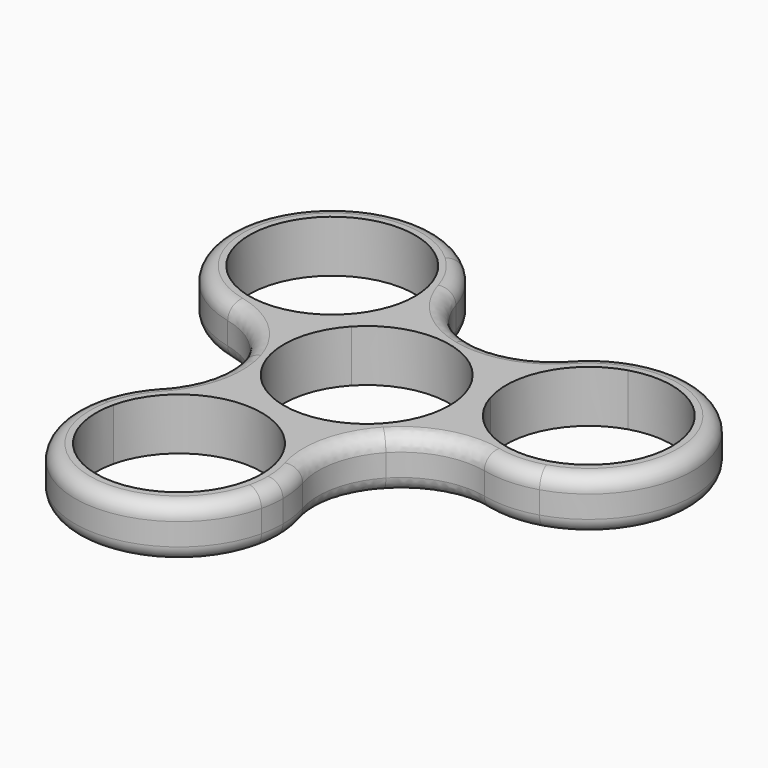
from build123d import *

# Parameters (mm, degrees)
F1_DEPTH = 7
F2_R     = 11.149
F3_R     = 2


# Not quite as in the source:
# - a fillet or chamfer is up to 0.001 mm smaller than in the source, because OpenCascade refuses the exact size


with BuildPart() as f1:
    # F0 (on Top) → F1 (new body)
    with BuildSketch(Plane.XY):
        with BuildLine():
            Line((-27.9345224248, 6.9415385111), (-25.9887218323, 9.0239313785))
            ThreePointArc((-25.9887218323, 9.0239313785), (-26.5231091537, 24.7833549146), (-10.7636856175, 25.317742236))
            Line((-10.7636856175, 25.317742236), (-8.8178850251, 27.4001351034))
            ThreePointArc((-8.8178850251, 27.4001351034), (-28.6055020211, 26.7291555071), (-27.9345224248, 6.9415385111))
        make_face()
        with BuildLine():
            ThreePointArc((-7.2262037249, 17.1708368072), (-8.0041138961, 13.0791070283), (-10.2292983588, 9.5583186329))
            ThreePointArc((-10.2292983588, 9.5583186329), (-7.8092966531, 11.6195906031), (-4.9866679164, 13.0817866934))
            ThreePointArc((-4.9866679164, 13.0817866934), (-4.5296608113, 15.1036528917), (-4.3762037249, 17.1708368072))
            ThreePointArc((-4.3762037249, 17.1708368072), (-4.3804864458, 17.5170994861), (-4.3933319882, 17.8631503155))
            ThreePointArc((-4.3933319882, 17.8631503155), (-7.4355430712, 22.246605973), (-8.8178850251, 27.4001351034))
            Line((-8.8178850251, 27.4001351034), (-10.7636856175, 25.317742236))
            ThreePointArc((-10.7636856175, 25.317742236), (-8.1487388167, 21.6117220288), (-7.2262037249, 17.1708368072))
        make_face()
        with BuildLine():
            Line((-10.2292982962, 9.5583186998), (-8.1469054287, 7.6125181074))
            ThreePointArc((-8.1469053912, 7.6125181475), (-6.2542997422, 10.166592106), (-4.9866679164, 13.0817866934))
            ThreePointArc((-4.9866679164, 13.0817866934), (-7.8092966531, 11.6195906031), (-10.2292983588, 9.5583186329))
        make_face()
        with BuildLine():
            ThreePointArc((-13.3895358085, 4.0890501138), (-10.5669070871, 5.5512461938), (-8.1469053912, 7.6125181475))
            Line((-8.1469054287, 7.6125181074), (-10.2292982962, 9.5583186998))
            ThreePointArc((-10.2292983588, 9.5583186329), (-12.1219039919, 7.0042446853), (-13.3895358085, 4.0890501138))
        make_face()
        with BuildLine():
            ThreePointArc((-13.3895358085, 4.0890501138), (-12.1219039919, 7.0042446853), (-10.2292983588, 9.5583186329))
            ThreePointArc((-10.2292983588, 9.5583186329), (-17.998334872, 6.0272415557), (-25.9887218323, 9.0239313785))
            Line((-25.9887218323, 9.0239313785), (-27.9345224248, 6.9415385111))
            ThreePointArc((-27.9345224248, 6.9415385111), (-22.699190816, 5.9114731141), (-18.11972388, 3.1731863583))
            ThreePointArc((-18.11972388, 3.1731863583), (-15.7149350018, 3.4261051335), (-13.3895358085, 4.0890501138))
        make_face()
        with BuildLine():
            ThreePointArc((-16.543965134, -21.9804963011), (-11.5813207167, -15.0379755337), (-3.1630976847, -13.6379915324))
            ThreePointArc((-3.1630976847, -13.6379915324), (-6.1582123683, -12.5728445638), (-8.8358256451, -10.8594744426))
            ThreePointArc((-8.8358256451, -10.8594744426), (-11.1358956381, -11.6055679238), (-13.2732759707, -12.7363122668))
            ThreePointArc((-13.2732759707, -12.7363122668), (-15.548354385, -17.5626721771), (-19.3202705541, -21.3365799911))
            Line((-19.3202705541, -21.3365799911), (-16.543965134, -21.9804963011))
        make_face()
        with BuildLine():
            Line((-3.1630976634, -13.6379915373), (-2.5191813534, -10.8616861172))
            ThreePointArc((-2.5191814257, -10.8616861004), (-5.6773771723, -10.4996785127), (-8.8358256451, -10.8594744426))
            ThreePointArc((-8.8358256451, -10.8594744426), (-6.1582123683, -12.5728445638), (-3.1630976847, -13.6379915324))
        make_face()
        with BuildLine():
            ThreePointArc((3.1535466283, -13.6402032119), (0.4759333083, -11.9268330695), (-2.5191814257, -10.8616861004))
            Line((-2.5191813534, -10.8616861172), (-3.1630976634, -13.6379915373))
            ThreePointArc((-3.1630976847, -13.6379915324), (-0.0049018926, -13.9999991418), (3.1535466283, -13.6402032119))
        make_face()
        with BuildLine():
            ThreePointArc((3.1535466283, -13.6402032119), (-0.0049018926, -13.9999991418), (-3.1630976847, -13.6379915324))
            ThreePointArc((-3.1630976847, -13.6379915324), (3.0473077962, -17.5630492175), (5.4677209832, -24.4996776545))
            ThreePointArc((5.4677209832, -24.4996776545), (5.3954080208, -25.7674906914), (5.1794071004, -27.0188590079))
            Line((5.1794071004, -27.0188590079), (7.9557125205, -27.662775318))
            ThreePointArc((7.9557125205, -27.662775318), (6.2301095174, -22.6138124491), (6.3118019427, -17.2787343688))
            ThreePointArc((6.3118019427, -17.2787343688), (4.8903734193, -15.3225854971), (3.1535466283, -13.6402032119))
        make_face()
        with BuildLine():
            ThreePointArc((5.1794071004, -27.0188590079), (-8.2014603702, -35.3613637717), (-16.543965134, -21.9804963011))
            Line((-16.543965134, -21.9804963011), (-19.3202705541, -21.3365799911))
            ThreePointArc((-19.3202705541, -21.3365799911), (-8.8453766803, -38.1376691918), (7.9557125205, -27.662775318))
            Line((7.9557125205, -27.662775318), (5.1794071004, -27.0188590079))
        make_face()
        with BuildLine():
            ThreePointArc((-8.8358256451, -10.8594744426), (-5.6773771723, -10.4996785127), (-2.5191814257, -10.8616861004))
            ThreePointArc((-2.5191814257, -10.8616861004), (-10.666086801, -3.249167948), (-8.1469053912, 7.6125181475))
            ThreePointArc((-8.1469053912, 7.6125181475), (-10.5669070871, 5.5512461938), (-13.3895358085, 4.0890501138))
            ThreePointArc((-13.3895358085, 4.0890501138), (-13.9999991418, 0.00490206), (-13.3923960635, -4.0796724964))
            ThreePointArc((-13.3923960635, -4.0796724964), (-11.6195907282, -7.809296467), (-8.8358256451, -10.8594744426))
        make_face()
        with BuildLine():
            ThreePointArc((10.6660867719, 3.2491680435), (11.0283581622, 1.6425030432), (11.15, 0))
            ThreePointArc((11.15, 0), (6.9366283994, -8.7295868429), (-2.5191814257, -10.8616861004))
            ThreePointArc((-2.5191814257, -10.8616861004), (0.4759333083, -11.9268330695), (3.1535466283, -13.6402032119))
            ThreePointArc((3.1535466283, -13.6402032119), (6.9957547845, -12.1268056385), (10.2292988758, -9.5583180795))
            ThreePointArc((10.2292988758, -9.5583180795), (12.5728447554, -6.1582119773), (13.8224935616, -2.2223122508))
            ThreePointArc((13.8224935616, -2.2223122508), (11.9316768823, 0.3330864457), (10.6660867719, 3.2491680435))
        make_face()
        with BuildLine():
            Line((13.3923959596, 4.0796728375), (10.6660867821, 3.2491680098))
            ThreePointArc((10.6660867719, 3.2491680435), (11.9316768823, 0.3330864457), (13.8224935616, -2.2223122508))
            ThreePointArc((13.8224935616, -2.2223122508), (13.955552835, -1.1146950565), (14, 0))
            ThreePointArc((14, 0), (13.8472658607, 2.0623356134), (13.392395974, 4.0796727904))
        make_face()
        with BuildLine():
            ThreePointArc((10.2359891802, 9.5511530981), (10.090973767, 6.3755869249), (10.6660867719, 3.2491680435))
            Line((10.6660867821, 3.2491680098), (13.3923959596, 4.0796728375))
            ThreePointArc((13.392395974, 4.0796727904), (12.1268058629, 6.9957543955), (10.2359891802, 9.5511530981))
        make_face()
        with BuildLine():
            ThreePointArc((-8.1469053912, 7.6125181475), (2.519181363, 10.861686115), (10.6660867719, 3.2491680435))
            ThreePointArc((10.6660867719, 3.2491680435), (10.090973767, 6.3755869249), (10.2359891802, 9.5511530981))
            ThreePointArc((10.2359891802, 9.5511530981), (7.0042446959, 12.1219039857), (3.1630975981, 13.6379915525))
            ThreePointArc((3.1630975981, 13.6379915525), (-0.9532539734, 13.9675089713), (-4.9866679164, 13.0817866934))
            ThreePointArc((-4.9866679164, 13.0817866934), (-6.2542997422, 10.166592106), (-8.1469053912, 7.6125181475))
        make_face()
        with BuildLine():
            ThreePointArc((10.2359891802, 9.5511530981), (12.1268058629, 6.9957543955), (13.392395974, 4.0796727904))
            ThreePointArc((13.392395974, 4.0796727904), (14.2189117048, 12.573394385), (20.8093147319, 17.9949276294))
            Line((20.8093147319, 17.9949276294), (19.9788099043, 20.7212368069))
            ThreePointArc((19.9788099043, 20.7212368069), (16.4690812987, 16.702339335), (11.8079219373, 14.1055480105))
            ThreePointArc((11.8079219373, 14.1055480105), (10.8245615825, 11.8964803637), (10.2359891802, 9.5511530981))
        make_face()
        with BuildLine():
            Line((19.9788099043, 20.7212368069), (20.8093147319, 17.9949276294))
            ThreePointArc((20.8093147319, 17.9949276294), (30.6952845578, 16.2884927186), (35.2084827418, 7.3288408473))
            ThreePointArc((35.2084827418, 7.3288408473), (33.018134613, 0.6920390313), (27.3076507516, -3.3372459348))
            Line((27.3076507516, -3.3372459348), (28.1381555792, -6.0635551123))
            ThreePointArc((28.1381555792, -6.0635551123), (35.3082698447, -1.0043632267), (38.0584827418, 7.3288408473))
            ThreePointArc((38.0584827418, 7.3288408473), (32.3916868157, 18.5786279503), (19.9788099043, 20.7212368069))
        make_face()
        with BuildLine():
            ThreePointArc((27.3076507516, -3.3372459348), (18.8139292041, -2.5107301896), (13.392395974, 4.0796727904))
            ThreePointArc((13.392395974, 4.0796727904), (13.8472658607, 2.0623356134), (14, 0))
            ThreePointArc((14, 0), (13.955552835, -1.1146950565), (13.8224935616, -2.2223122508))
            ThreePointArc((13.8224935616, -2.2223122508), (15.6186644664, -3.8411845546), (17.6666079589, -5.1268380487))
            ThreePointArc((17.6666079589, -5.1268380487), (22.9838974562, -4.6839337959), (28.1381555792, -6.0635551123))
            Line((28.1381555792, -6.0635551123), (27.3076507516, -3.3372459348))
        make_face()
        with BuildLine():
            ThreePointArc((19.9788099043, 20.7212368069), (15.2487740483, 18.2095132868), (11.8079219373, 14.1055480105))
            ThreePointArc((11.8079219373, 14.1055480105), (16.4690812987, 16.702339335), (19.9788099043, 20.7212368069))
        make_face()
        with BuildLine():
            ThreePointArc((-8.8178850251, 27.4001351034), (-7.4355430712, 22.246605973), (-4.3933319882, 17.8631503155))
            ThreePointArc((-4.3933319882, 17.8631503155), (-5.6763835882, 23.0627438411), (-8.8178850251, 27.4001351034))
        make_face()
        with BuildLine():
            ThreePointArc((-27.9345224248, 6.9415385111), (-23.3942881211, 4.101069059), (-18.11972388, 3.1731863583))
            ThreePointArc((-18.11972388, 3.1731863583), (-22.699190816, 5.9114731141), (-27.9345224248, 6.9415385111))
        make_face()
        with BuildLine():
            ThreePointArc((-19.3202705541, -21.3365799911), (-15.548354385, -17.5626721771), (-13.2732759707, -12.7363122668))
            ThreePointArc((-13.2732759707, -12.7363122668), (-17.1347302533, -16.4472643096), (-19.3202705541, -21.3365799911))
        make_face()
        with BuildLine():
            ThreePointArc((28.1381555792, -6.0635551123), (22.9838974562, -4.6839337959), (17.6666079589, -5.1268380487))
            ThreePointArc((17.6666079589, -5.1268380487), (22.8111138415, -6.6154795315), (28.1381555792, -6.0635551123))
        make_face()
        with BuildLine():
            ThreePointArc((8.3177209832, -24.4996776545), (7.8069228393, -20.7524876029), (6.3118019427, -17.2787343688))
            ThreePointArc((6.3118019427, -17.2787343688), (6.2301095174, -22.6138124491), (7.9557125205, -27.662775318))
            ThreePointArc((7.9557125205, -27.662775318), (8.2269244385, -26.091550526), (8.3177209832, -24.4996776545))
        make_face()
    extrude(amount=F1_DEPTH)

    # F2 (radius 11.15 in the source; OpenCascade refuses exactly that, so slightly less here)
    f2_edges = [f1.edges().sort_by_distance(p)[0] for p in [
        (-13.389536, 4.08905, 3.5),
        (-8.835826, -10.859474, 3.5),
        (10.235989, 9.551153, 3.5),
        (-4.986668, 13.081787, 3.5),
        (13.822494, -2.222312, 3.5),
        (3.153547, -13.640203, 3.5),
    ]]
    fillet(f2_edges, radius=F2_R)

    # F3
    f3_edges = [f1.edges().sort_by_distance(p)[0] for p in [
        (-8.845377, -38.137669, 7),
        (-8.845377, -38.137669, 0),
    ]]
    fillet(f3_edges, radius=F3_R)


solid = f1.part
